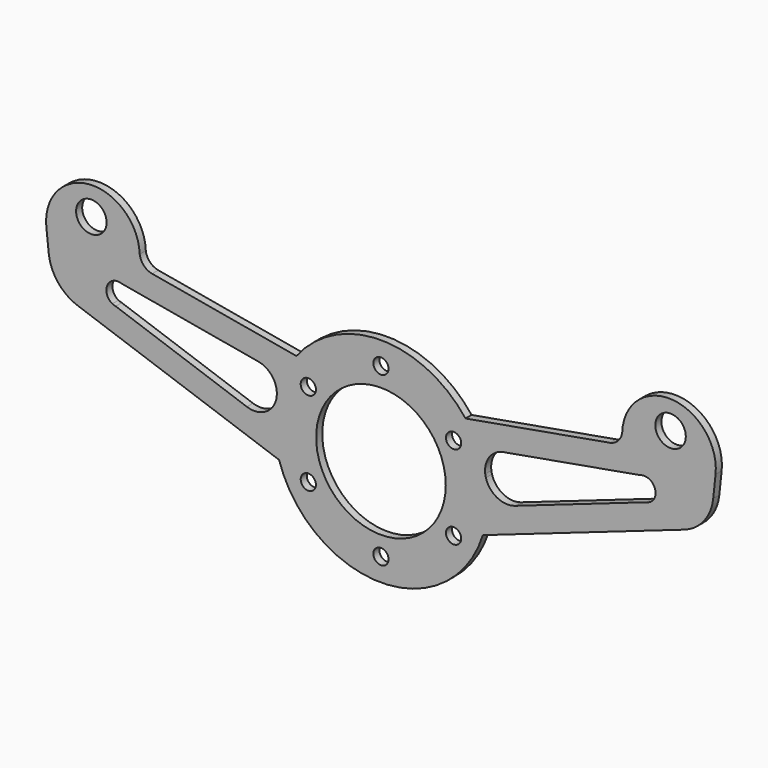
from build123d import *

# Parameters (mm, degrees)
F0_R     = 6.35
F0_R_2   = 3.175
F0_R_3   = 26.9875
F1_DEPTH = 3.175


# Not quite as in the source:
# - a feature names something its author has since deleted; it is built from what else it names


with BuildPart() as f1:
    # F0 (on Front) → F1 (new body)
    with BuildSketch(Plane.XZ):
        with BuildLine():
            ThreePointArc((-43.4258934254, 9.4865315159), (-40.2925849359, 18.769925391), (-35.2015661866, 27.1413381765))
            Line((-35.2015661866, 27.1413381765), (-95.2689163392, 37.7723748329))
            ThreePointArc((-95.2689163392, 37.7723748329), (-98.7721627257, 39.6581308221), (-100.4657668126, 43.2582025009))
            ThreePointArc((-100.4657668126, 43.2582025009), (-121.3252913638, 62.0407471137), (-139.3392654958, 40.5140083313))
            Line((-139.3392654958, 40.5140083313), (-138.3529874387, 31.3088718833))
            ThreePointArc((-138.3529874387, 31.3088718833), (-134.5315509232, 21.8873221018), (-126.2516022963, 15.9872010809))
            Line((-126.2516022963, 15.9872010809), (-42.4180155898, -13.285874206))
            ThreePointArc((-42.4180155899, -13.285874206), (-44.3727417421, -2.6195973531), (-43.6866122567, 8.2025855396))
            ThreePointArc((-43.6866122567, 8.2025855396), (-48.388636459, 2.3785824935), (-55.8537619567, 1.8309107075))
            Line((-55.8537619567, 1.8309107075), (-110.4577448757, 20.8975708106))
            ThreePointArc((-110.4577448757, 20.8975708106), (-111.1735466188, 21.086419267), (-111.8513183434, 21.3841798493))
            ThreePointArc((-111.8513183434, 21.3841798493), (-114.2200668687, 26.7082159188), (-109.6486913125, 30.321919721))
            ThreePointArc((-109.6486913125, 30.321919721), (-108.7795274506, 30.2493985469), (-107.9382701007, 30.0192003476))
            Line((-107.9382701007, 30.0192003476), (-51.5976439548, 20.0477389749))
            ThreePointArc((-51.5976439548, 20.0477389749), (-51.1132512592, 19.9749597914), (-50.6333036668, 19.8770649411))
            ThreePointArc((-50.6333036668, 19.8770649411), (-45.0232212062, 16.073525101), (-43.4258934254, 9.4865315159))
        make_face()
        with Locations((-120.6001266837, 50.3768287599)):
            Circle(F0_R, mode=Mode.SUBTRACT)
        with BuildLine():
            ThreePointArc((35.2015661866, 27.1413381765), (0, 44.45), (-35.2015661866, 27.1413381765))
            ThreePointArc((-35.2015661866, 27.1413381765), (-40.2925849359, 18.769925391), (-43.4258934254, 9.4865315159))
            ThreePointArc((-43.4258934254, 9.4865315159), (-43.533872992, 8.8400140623), (-43.6866122567, 8.2025855396))
            ThreePointArc((-43.6866122567, 8.2025855396), (-44.3727417421, -2.6195973531), (-42.4180155899, -13.285874206))
            ThreePointArc((-42.4180155899, -13.285874206), (0, -44.45), (42.4180155899, -13.285874206))
            ThreePointArc((42.4180155899, -13.285874206), (43.9390674285, -6.7201825508), (44.45, 0))
            ThreePointArc((44.45, 0), (44.2587415931, 4.1190159741), (43.6866122567, 8.2025855396))
            ThreePointArc((43.6866122567, 8.2025855396), (43.533872992, 8.8400140623), (43.4258934254, 9.4865315159))
            ThreePointArc((43.4258934254, 9.4865315159), (40.2925849359, 18.769925391), (35.2015661866, 27.1413381765))
        make_face()
        with Locations((0, -34.925)):
            Circle(F0_R_2, mode=Mode.SUBTRACT)
        with Locations((-30.2459372272, -17.4625)):
            Circle(F0_R_2, mode=Mode.SUBTRACT)
        Circle(F0_R_3, mode=Mode.SUBTRACT)
        with Locations((30.2459372272, -17.4625)):
            Circle(F0_R_2, mode=Mode.SUBTRACT)
        with Locations((-30.2459372272, 17.4625)):
            Circle(F0_R_2, mode=Mode.SUBTRACT)
        with Locations((0, 34.925)):
            Circle(F0_R_2, mode=Mode.SUBTRACT)
        with Locations((30.2459372272, 17.4625)):
            Circle(F0_R_2, mode=Mode.SUBTRACT)
        with BuildLine():
            Line((95.2689163392, 37.7723748329), (35.2015661866, 27.1413381765))
            ThreePointArc((35.2015661866, 27.1413381765), (40.2925849359, 18.769925391), (43.4258934254, 9.4865315159))
            ThreePointArc((43.4258934254, 9.4865315159), (45.0232212062, 16.073525101), (50.6333036668, 19.8770649411))
            ThreePointArc((50.6333036668, 19.8770649411), (51.1132512592, 19.9749597914), (51.5976439548, 20.0477389749))
            Line((51.5976439548, 20.0477389749), (107.9382701008, 30.0192003476))
            ThreePointArc((107.9382701008, 30.0192003476), (108.7795274506, 30.2493985469), (109.6486913125, 30.321919721))
            ThreePointArc((109.6486913125, 30.321919721), (114.2200668687, 26.7082159188), (111.8513183434, 21.3841798493))
            ThreePointArc((111.8513183434, 21.3841798493), (111.1735466188, 21.086419267), (110.4577448757, 20.8975708106))
            Line((110.4577448757, 20.8975708106), (55.8537619567, 1.8309107075))
            ThreePointArc((55.8537619567, 1.8309107075), (48.388636459, 2.3785824935), (43.6866122567, 8.2025855396))
            ThreePointArc((43.6866122567, 8.2025855396), (44.2587415931, 4.1190159741), (44.45, 0))
            ThreePointArc((44.45, 0), (43.9390674285, -6.7201825508), (42.4180155899, -13.285874206))
            Line((42.4180155898, -13.285874206), (126.2516022963, 15.9872010809))
            ThreePointArc((126.2516022963, 15.9872010809), (134.5315509232, 21.8873221018), (138.3529874387, 31.3088718833))
            Line((138.3529874387, 31.3088718833), (139.3392654958, 40.5140083313))
            ThreePointArc((139.3392654958, 40.5140083313), (121.3252913638, 62.0407471137), (100.4657668126, 43.2582025009))
            ThreePointArc((100.4657668126, 43.2582025009), (98.7721627257, 39.6581308221), (95.2689163392, 37.7723748329))
        make_face()
        with Locations((120.6001266837, 50.3768287599)):
            Circle(F0_R, mode=Mode.SUBTRACT)
    extrude(amount=F1_DEPTH)


solid = f1.part
